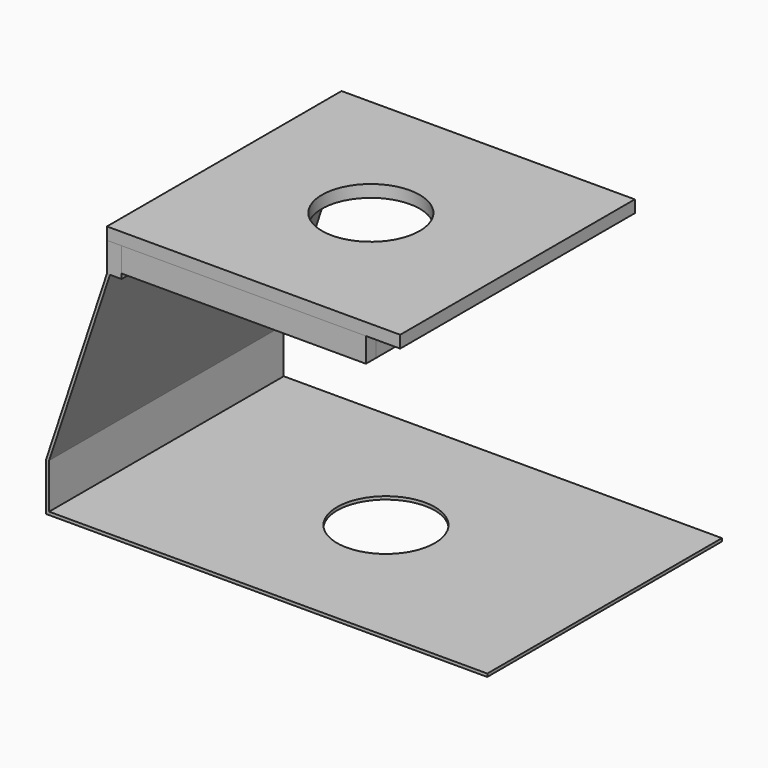
from build123d import *

# Parameters (mm, degrees)
F0_W      = 76.2
F0_H      = 76.2
F1_DEPTH  = 3.175
F2_R      = 12.7
F3_DEPTH  = 3.176
F4_W      = 76.2
F4_H      = 7.62
F5_DEPTH  = 3.81
F7_W      = 3.175
F7_H      = 6.35
F8_DEPTH  = 63.5
F12_DEPTH = 76.2
F13_DEPTH = 76.2
F14_R     = 12.7
F15_DEPTH = 0.79475
F16_W     = 3.175
F16_H     = 6.35
F17_DEPTH = 57.15


# Not quite as in the source:
# - a feature names something its author has since deleted; it is built from what else it names


with BuildPart() as f1:
    # F0 (on Top) → F1 (new body)
    with BuildSketch(Plane.XY):
        with Locations((38.1, 38.1)):
            Rectangle(F0_W, F0_H)
    extrude(amount=F1_DEPTH)

    # F2 (on face) → F3 (cut, through all)
    with BuildSketch(Plane.XY.offset(3.175)):
        with Locations((38.1, 38.1)):
            Circle(F2_R)
    extrude(amount=-F3_DEPTH, mode=Mode.SUBTRACT)


with BuildPart() as f5:
    # F4 (on face) → F5 (new body)
    with BuildSketch(Plane(origin=(0, 0, 0), x_dir=(0, -1, 0), z_dir=(-1, 0, 0))):
        with Locations((-38.1, -3.81)):
            Rectangle(F4_W, F4_H)
    extrude(amount=-F5_DEPTH)


with BuildPart() as f8:
    # F7 (on face) → F8 (new body)
    with BuildSketch(Plane.YZ.offset(3.81)):
        with Locations((1.5875, -3.175)):
            Rectangle(F7_W, F7_H)
    extrude(amount=F8_DEPTH)


with BuildPart() as f12:
    # F11 (on face) → F12 (new body)
    with BuildSketch(Plane(origin=(0, 76.2, 0), x_dir=(-1, 0, 0), z_dir=(0, 1, 0))):
        Polygon((15.81023, -55.2641394734), (0, -7.62), (-0.79375, -7.62), (15.01648, -55.2641394734), (15.01648, -66.9532194734), (15.01648, -67.7469694734), (15.81023, -67.7469694734), align=None)
    extrude(amount=-F12_DEPTH)


with BuildPart() as f13:
    # F11 (on face) → F13 (new body)
    with BuildSketch(Plane(origin=(0, 76.2, 0), x_dir=(-1, 0, 0), z_dir=(0, 1, 0))):
        Polygon((15.01648, -67.7469694734), (15.01648, -66.9532194734), (-98.83648, -66.9532194734), (-98.82632, -67.7469694734), align=None)
    extrude(amount=-F13_DEPTH)

    # F14 (on face) → F15 (cut, through all)
    with BuildSketch(Plane.XY.offset(-66.9532194734)):
        with Locations((42.0243, 38.1)):
            Circle(F14_R)
    extrude(amount=-F15_DEPTH, mode=Mode.SUBTRACT)


with BuildPart() as f17:
    # F16 (on face) → F17 (new body)
    with BuildSketch(Plane(origin=(0, 3.175, 0), x_dir=(-1, 0, 0), z_dir=(0, 1, 0))):
        with Locations((-65.7225, -3.175)):
            Rectangle(F16_W, F16_H)
    extrude(amount=F17_DEPTH)


solid = Compound([f1.part, f5.part, f8.part, f12.part, f13.part, f17.part])
